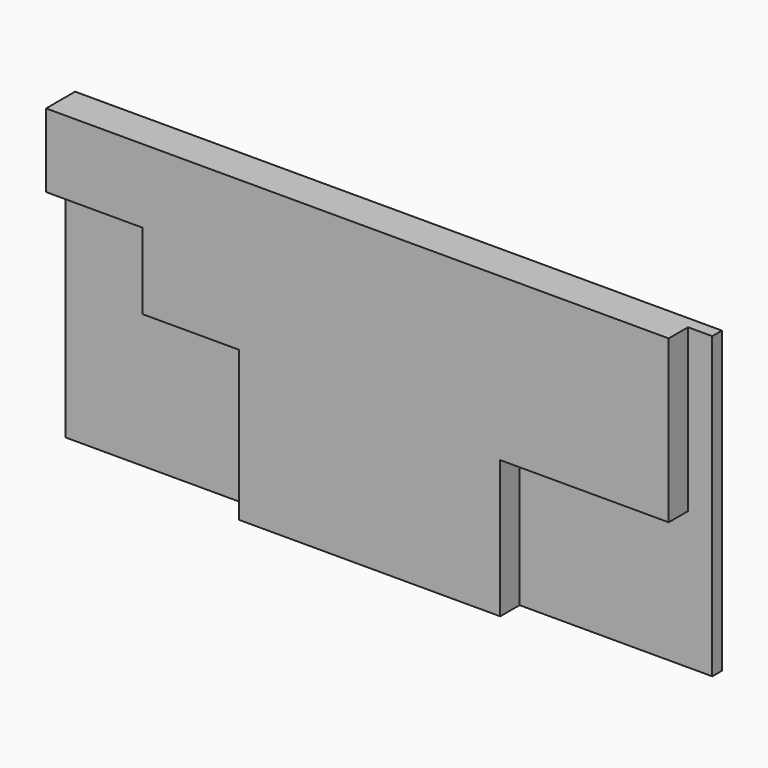
from build123d import *

# Parameters (mm, degrees)
F1_DEPTH = 10
F2_W     = 69.6255117655
F2_H     = 56.8695068359
F3_DEPTH = 5
F4_W     = 5
F4_H     = 123.7891986966
F5_DEPTH = 10


with BuildPart() as f1:
    # F0 (on Front) → F1 (new body)
    with BuildSketch(Plane.XZ):
        Polygon((126.4532655478, 59.8521605134), (-130.8932900429, 59.8521605134), (-130.8932900429, 29.4098556042), (-91.0648927093, 29.4098556042), (-91.0648927093, -2.0424388349), (-51.2364953756, -2.0424388349), (-51.2364953756, -63.9370381832), (56.8277537823, -63.9370381832), (56.8277537823, -7.0675313473), (126.4532655478, -7.0675313473), align=None)
    extrude(amount=F1_DEPTH)

    # F2 (on face) → F3 (join)
    with BuildSketch(Plane(origin=(0, 0, 0), x_dir=(-1, 0, 0), z_dir=(0, 1, 0))):
        Polygon((51.2364953756, -63.9370381832), (130.8932900429, -63.9370381832), (130.8932900429, 29.4098556042), (91.0648927093, 29.4098556042), (91.0648927093, -2.0424388349), (51.2364953756, -2.0424388349), align=None)
        with Locations((-91.640509665, -35.5022847652)):
            Rectangle(F2_W, F2_H)
        Polygon((-56.8277537823, -63.9370381832), (51.2364953756, -63.9370381832), (51.2364953756, -2.0424388349), (91.0648927093, -2.0424388349), (91.0648927093, 29.4098556042), (130.8932900429, 29.4098556042), (130.8932900429, 59.8521605134), (-126.4532655478, 59.8521605134), (-126.4532655478, -7.0675313473), (-56.8277537823, -7.0675313473), align=None)
    extrude(amount=F3_DEPTH)

    # F4 (on face) → F5 (join)
    with BuildSketch(Plane.YZ.offset(126.4532655478)):
        with Locations((2.5, -2.0424388349)):
            Rectangle(F4_W, F4_H)
    extrude(amount=F5_DEPTH)


solid = f1.part
